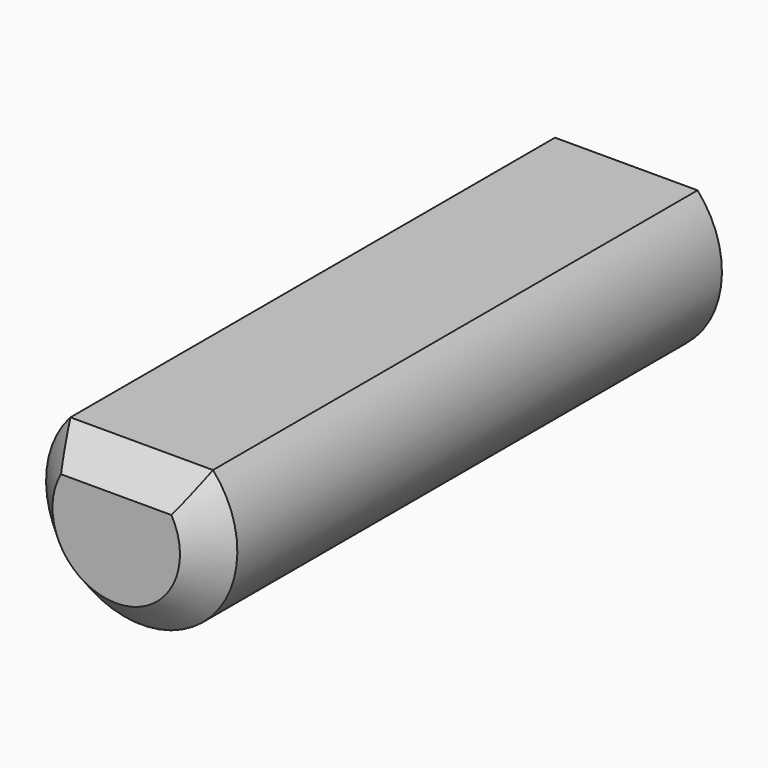
from build123d import *

# Parameters (mm, degrees)
F1_DEPTH = 10
F2_SIZE  = 0.49999


# Not quite as in the source:
# - a fillet or chamfer is up to 0.001 mm smaller than in the source, because OpenCascade refuses the exact size
# - a feature names something its author has since deleted; it is built from what else it names


with BuildPart() as f1:
    # F0 (on Front) → F1 (new body)
    with BuildSketch(Plane.XZ):
        with BuildLine():
            Line((1.1180339887, 1), (-1.1180339887, 1))
            ThreePointArc((-1.1180339887, 1), (0, -1.5), (1.1180339887, 1))
        make_face()
    extrude(amount=F1_DEPTH)

    # F2 (size 0.5 in the source; OpenCascade refuses exactly that, so slightly less here)
    f2_edges = [f1.edges().sort_by_distance(p)[0] for p in [
        (0, -10, 1),
        (0, -10, -1.5),
    ]]
    chamfer(f2_edges, length=F2_SIZE)


solid = f1.part
